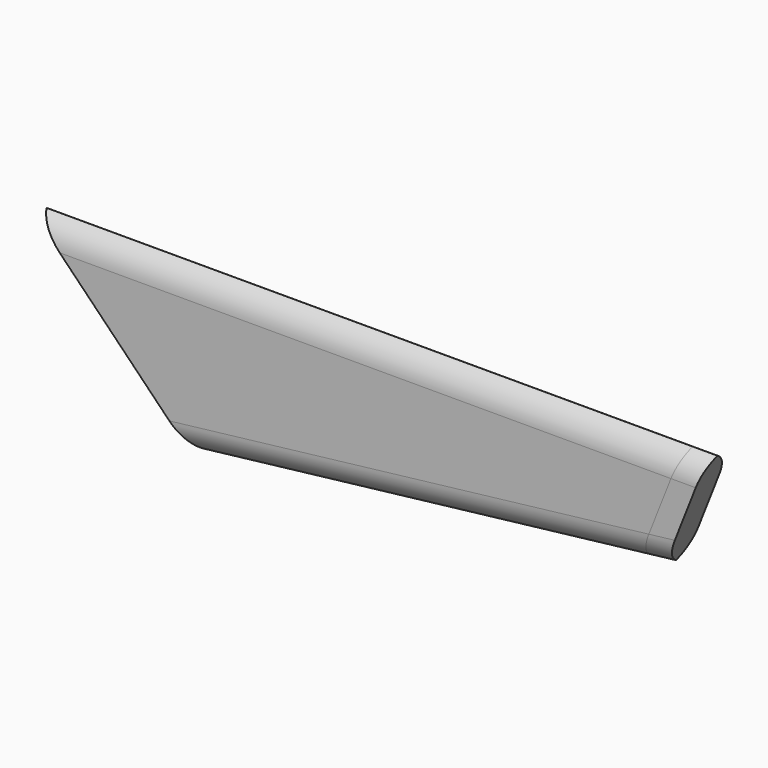
from build123d import *

# Parameters (mm, degrees)
F1_DEPTH    = 2.5
F2_T1_DEPTH = 135.7792679391
F2_T3_DEPTH = 100.5448710702
F3_DEPTH    = 2.5
F4_T1_DEPTH = 29.2207320609
F4_T3_DEPTH = 29.4551289298


# Not quite as in the source:
# - a fillet or chamfer that OpenCascade refuses, or shapes differently, is made with other operations: its cross-section is extruded or revolved along the edge and cut away or added


with BuildPart() as f1:
    # F0 (on Front) → F1 (new body, symmetric)
    with BuildSketch(Plane.XZ):
        Polygon((63.2162865844, 0), (-47.5629813547, 0), (-19.6151699151, -28.6167754252), (55.4160096247, -19.8219109079), align=None)
    extrude(amount=F1_DEPTH, both=True)

    # F2: fillet of radius 5 on 4 edges, made by hand

    # F2_s2 → F2_t1 (cut)
    with BuildSketch(Plane.YZ.offset(-60.0629813547)):
        with BuildLine():
            ThreePointArc((2.5, 0), (-1.0355339059, -1.4644660941), (-2.5, -5))
            Line((-2.5, -5), (-2.5, 0))
            Line((-2.5, 0), (2.5, 0))
        make_face()
        with BuildLine():
            ThreePointArc((-2.5, 0), (1.0355339059, -1.4644660941), (2.5, -5))
            Line((2.5, -5), (2.5, 0))
            Line((2.5, 0), (-2.5, 0))
        make_face()
    extrude(amount=F2_T1_DEPTH, mode=Mode.SUBTRACT)

    # F2_s4 → F2_t3 (cut)
    with BuildSketch(Plane(origin=(-35.073204722, 0, -4.1111453346), x_dir=(0, 1, 0), z_dir=(0.9932001799, 0, 0.1164190817))):
        with BuildLine():
            ThreePointArc((2.5, -26.1386064324), (-1.0355339059, -24.6741403384), (-2.5, -21.1386064324))
            Line((-2.5, -21.1386064324), (-2.5, -26.1386064324))
            Line((-2.5, -26.1386064324), (2.5, -26.1386064324))
        make_face()
        with BuildLine():
            ThreePointArc((-2.5, -26.1386064324), (1.0355339059, -24.6741403384), (2.5, -21.1386064324))
            Line((2.5, -21.1386064324), (2.5, -26.1386064324))
            Line((2.5, -26.1386064324), (-2.5, -26.1386064324))
        make_face()
    extrude(amount=F2_T3_DEPTH, mode=Mode.SUBTRACT)


with BuildPart() as f3:
    # F0 (on Front) → F3 (new body, symmetric)
    with BuildSketch(Plane.XZ):
        Polygon((67.4370186453, 0), (63.2162865844, 0), (55.4160096247, -19.8219109079), (59.8408444794, -19.3032488891), align=None)
    extrude(amount=F3_DEPTH, both=True)

    # F4: fillet of radius 5 on 4 edges, made by hand

    # F4_s2 → F4_t1 (cut)
    with BuildSketch(Plane.YZ.offset(50.7162865844)):
        with BuildLine():
            ThreePointArc((-2.5, -5), (-1.0355339059, -1.4644660941), (2.5, 0))
            Line((2.5, 0), (-2.5, 0))
            Line((-2.5, 0), (-2.5, -5))
        make_face()
        with BuildLine():
            ThreePointArc((-2.5, 0), (1.0355339059, -1.4644660941), (2.5, -5))
            Line((2.5, -5), (2.5, 0))
            Line((2.5, 0), (-2.5, 0))
        make_face()
    extrude(amount=F4_T1_DEPTH, mode=Mode.SUBTRACT)

    # F4_s4 → F4_t3 (cut)
    with BuildSketch(Plane(origin=(39.9579748177, 0, 4.6837191826), x_dir=(0, 1, 0), z_dir=(0.9932001799, 0, 0.1164190817))):
        with BuildLine():
            ThreePointArc((2.5, -26.1386064324), (-1.0355339059, -24.6741403384), (-2.5, -21.1386064324))
            Line((-2.5, -21.1386064324), (-2.5, -26.1386064324))
            Line((-2.5, -26.1386064324), (2.5, -26.1386064324))
        make_face()
        with BuildLine():
            ThreePointArc((-2.5, -26.1386064324), (1.0355339059, -24.6741403384), (2.5, -21.1386064324))
            Line((2.5, -21.1386064324), (2.5, -26.1386064324))
            Line((2.5, -26.1386064324), (-2.5, -26.1386064324))
        make_face()
    extrude(amount=F4_T3_DEPTH, mode=Mode.SUBTRACT)


solid = Compound([f1.part, f3.part])
